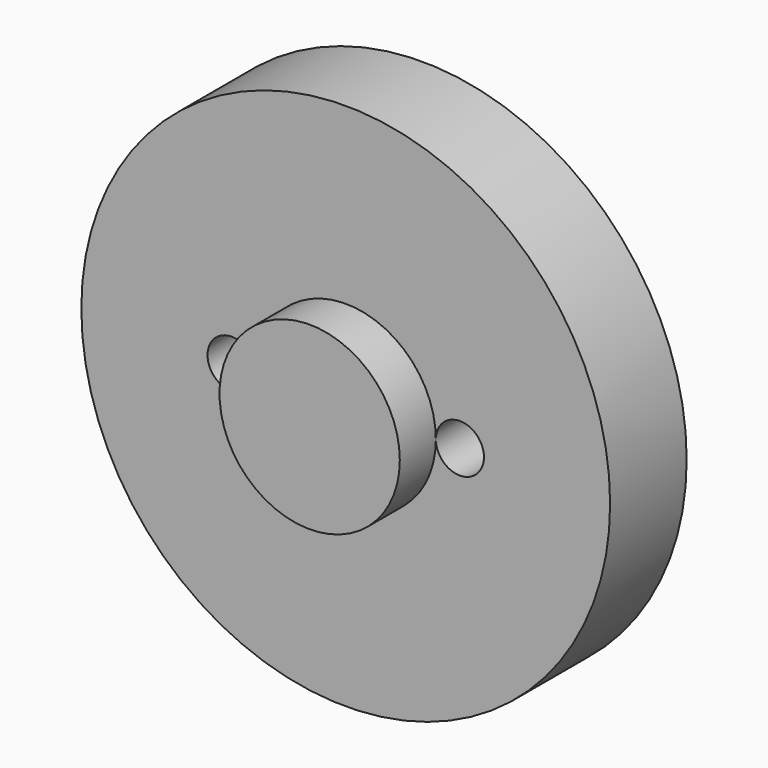
from build123d import *

# Parameters (mm, degrees)
F0_R     = 17.6
F0_R_2   = 1.6
F0_R_3   = 4.45
F1_DEPTH = 6.37
F2_R     = 3.95
F2_R_2   = 2.38125
F3_DEPTH = 6.37
F2_R_3   = 4.45
F4_DEPTH = 3
F5_SIZE  = 1


with BuildPart() as f1:
    # F0 (on Front) → F1 (new body)
    with BuildSketch(Plane.XZ):
        Circle(F0_R)
        with Locations((-7.6, 0)):
            Circle(F0_R_2, mode=Mode.SUBTRACT)
        Circle(F0_R_3, mode=Mode.SUBTRACT)
        with Locations((7.6, 0)):
            Circle(F0_R_2, mode=Mode.SUBTRACT)
    extrude(amount=F1_DEPTH)


with BuildPart() as f3:
    # F2 (on face) → F3 (new body, through all)
    with BuildSketch(Plane.XZ.offset(6.37)):
        Circle(F2_R)
        Circle(F2_R_2, mode=Mode.SUBTRACT)
    extrude(amount=-F3_DEPTH)

    # F2 (on face) → F4 (join)
    with BuildSketch(Plane.XZ.offset(6.37)):
        with BuildLine():
            ThreePointArc((-6, 0), (0, -6), (6, 0))
            ThreePointArc((6, 0), (0, 6), (-6, 0))
        make_face()
        Circle(F2_R_3, mode=Mode.SUBTRACT)
        Circle(F2_R_3)
        Circle(F2_R, mode=Mode.SUBTRACT)
        Circle(F2_R)
        Circle(F2_R_2, mode=Mode.SUBTRACT)
        Circle(F2_R_2)
    extrude(amount=F4_DEPTH)

    # F5
    f5_edges = [f3.edges().sort_by_distance(p)[0] for p in [
        (-2.38125, 0, 0),
    ]]
    chamfer(f5_edges, length=F5_SIZE)


solid = Compound([f1.part, f3.part])
